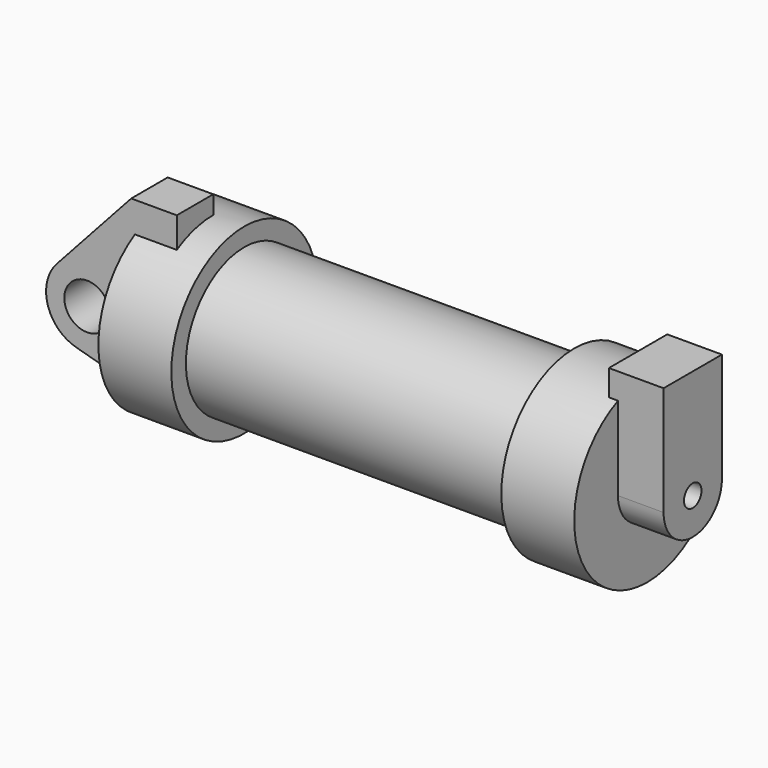
from build123d import *

# Parameters (mm, degrees)
F0_W     = 5.842
F0_H     = 12.7
F0_R     = 3.175
F2_DEPTH = 6.35
F3_R     = 1.524
F4_DEPTH = 6.35
F5_DEPTH = 7.62


with BuildPart() as f1:
    # F0 (on Front) → F1 (revolve)
    with BuildSketch(Plane.XZ):
        Polygon((5.842, 12.7), (5.842, 0), (66.294, 0), (66.294, 12.7), (56.134, 12.7), (56.134, 10.16), (10.16, 10.16), (10.16, 12.7), align=None)
        with Locations((2.921, 6.35)):
            Rectangle(F0_W, F0_H)
    revolve(axis=Axis((33.147, 0, 0), (-1, 0, 0)))

    # F0 (on Front) → F2 (join)
    with BuildSketch(Plane.XZ):
        with BuildLine():
            Line((-0.9398, 0), (0, 0))
            Line((0, 0), (0, 12.7))
            Line((0, 12.7), (5.842, 12.7))
            Line((5.842, 12.7), (5.842, 15.24))
            Line((5.842, 15.24), (-0.508, 15.24))
            Line((-0.508, 15.24), (-10.8806298187, 3.8475430269))
            ThreePointArc((-10.8806298187, 3.8475430269), (-4.5919612295, 5.3297205562), (-0.9398, 0))
        make_face()
        with BuildLine():
            Line((5.842, 0), (0, 0))
            Line((0, 0), (-0.9398, 0))
            ThreePointArc((-0.9398, 0), (-3.1957909266, -4.5493385486), (-8.1826630726, -5.5069827884))
            Line((-8.1826630726, -5.5069827884), (5.842, -9.398))
            Line((5.842, -9.398), (5.842, 0))
        make_face()
        with Locations((2.921, 6.35)):
            Rectangle(F0_W, F0_H)
        with BuildLine():
            ThreePointArc((-8.1826630726, -5.5069827884), (-3.1957909266, -4.5493385486), (-0.9398, 0))
            ThreePointArc((-0.9398, 0), (-4.5919612295, 5.3297205562), (-10.8806298187, 3.8475430269))
            ThreePointArc((-10.8806298187, 3.8475430269), (-12.1459778134, -1.5837270034), (-8.1826630726, -5.5069827884))
        make_face()
        with Locations((-6.6548, 0)):
            Circle(F0_R, mode=Mode.SUBTRACT)
    extrude(amount=F2_DEPTH)

    # F3 (on face) → F4 (join)
    with BuildSketch(Plane.YZ.offset(66.294)):
        with BuildLine():
            ThreePointArc((-5.08, 11.6397422652), (0, 12.7), (5.08, 11.6397422652))
            Line((5.08, 11.6397422652), (5.08, 15.24))
            Line((5.08, 15.24), (-5.08, 15.24))
            Line((-5.08, 15.24), (-5.08, 11.6397422652))
        make_face()
        with BuildLine():
            ThreePointArc((-5.08, 0), (0, 5.08), (5.08, 0))
            Line((5.08, 0), (5.08, 11.6397422652))
            ThreePointArc((5.08, 11.6397422652), (0, 12.7), (-5.08, 11.6397422652))
            Line((-5.08, 11.6397422652), (-5.08, 0))
        make_face()
        with BuildLine():
            ThreePointArc((-5.08, 0), (0, -5.08), (5.08, 0))
            ThreePointArc((5.08, 0), (0, 5.08), (-5.08, 0))
        make_face()
        Circle(F3_R, mode=Mode.SUBTRACT)
    extrude(amount=F4_DEPTH)

    # F5 (add): a face of the model
    f5_faces = [f1.faces().sort_by_distance(p)[0] for p in [
        (72.644, 0, 5.8085929676),
    ]]
    extrude(f5_faces, amount=-F5_DEPTH)


solid = f1.part
